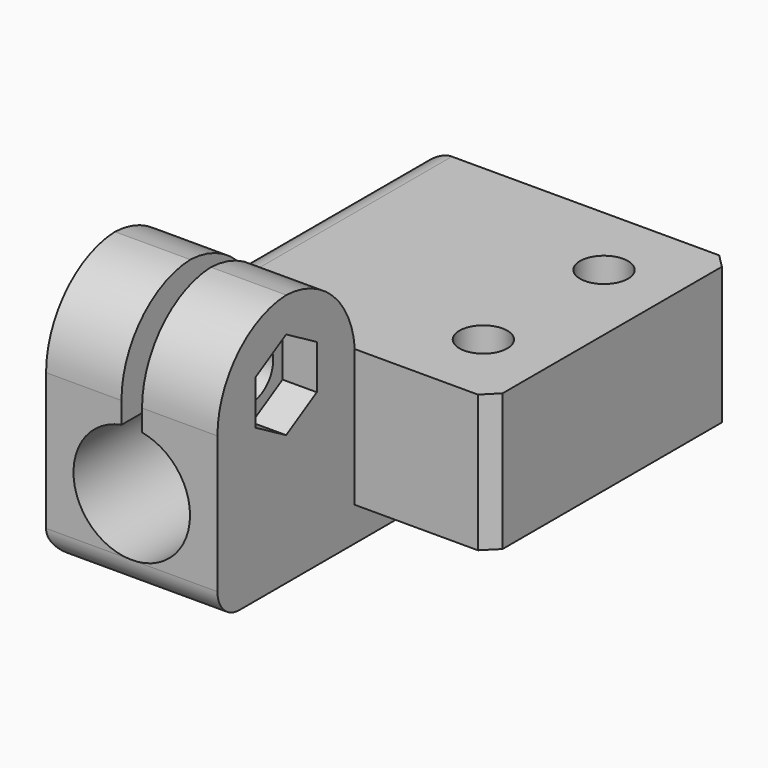
from build123d import *

# Parameters (mm, degrees)
F0_W         = 25
F0_H         = 44
F0_H_2       = 25
F1_DEPTH     = 25
F0_W_2       = 20
F0_R         = 3.5
F2_DEPTH     = 25
F3_R         = 8.5
F4_DEPTH     = 69.001
F5_W         = 11
F5_H         = 25.0466239899
F6_DEPTH     = 12
F5_W_2       = 3
F5_H_2       = 6.9533760101
F7_DEPTH     = 4.1343997347
F9_T1_DEPTH  = 76
F9_T3_DEPTH  = 76
F9_T5_DEPTH  = 75.8074069841
F9_T7_DEPTH  = 75.8074069841
F10_DEPTH    = 5
F8_R         = 3.9
F11_DEPTH    = 25.001
F12_DEPTH    = 25.001
F13_DEPTH    = 5
F14_R        = 3.99999
F15_T1_DEPTH = 30.2867319519


# Not quite as in the source:
# - a fillet or chamfer that OpenCascade refuses, or shapes differently, is made with other operations: its cross-section is extruded or revolved along the edge and cut away or added
# - a fillet or chamfer is up to 0.001 mm smaller than in the source, because OpenCascade refuses the exact size
# - a feature names something its author has since deleted; it is built from what else it names


with BuildPart() as f1:
    # F0 (on Top) → F1 (new body)
    with BuildSketch(Plane.XY):
        Rectangle(F0_W, F0_H)
        with Locations((0, -34.5)):
            Rectangle(F0_W, F0_H_2)
    extrude(amount=F1_DEPTH)

    # F0 (on Top) → F2 (join)
    with BuildSketch(Plane.XY):
        with Locations((22.5, 0)):
            Rectangle(F0_W_2, F0_H)
        with Locations((22.5, -11)):
            Circle(F0_R, mode=Mode.SUBTRACT)
        with Locations((22.5, 11)):
            Circle(F0_R, mode=Mode.SUBTRACT)
    extrude(amount=F2_DEPTH)

    # F3 (on face) → F4 (cut, through all)
    with BuildSketch(Plane.XZ.offset(47)):
        with Locations((0, 12.5)):
            Circle(F3_R)
    extrude(amount=-F4_DEPTH, mode=Mode.SUBTRACT)

    # F5 (on face) → F6 (join)
    with BuildSketch(Plane.XY.offset(25)):
        with Locations((-7, -34.476688005)):
            Rectangle(F5_W, F5_H)
        Polygon((12.5, -22), (12.5, -21.9533760101), (1.5, -21.9533760101), (1.5, -47), (12.5, -47), align=None)
    extrude(amount=F6_DEPTH)

    # F5 (on face) → F7 (cut, through all)
    with BuildSketch(Plane.XY.offset(25)):
        with Locations((0, -34.476688005)):
            Rectangle(F5_W_2, F5_H)
        with Locations((0, -18.476688005)):
            Rectangle(F5_W_2, F5_H_2)
    extrude(amount=-F7_DEPTH, mode=Mode.SUBTRACT)

    # F9: fillet of radius 13 on 4 edges, made by hand

    # F9_s2 → F9_t1 (cut)
    with BuildSketch(Plane.YZ.offset(-45)):
        with BuildLine():
            ThreePointArc((-34, 37), (-43.1923881554, 33.1923881554), (-47, 24))
            Line((-47, 24), (-47, 37))
            Line((-47, 37), (-34, 37))
        make_face()
    extrude(amount=F9_T1_DEPTH, mode=Mode.SUBTRACT)

    # F9_s4 → F9_t3 (cut)
    with BuildSketch(Plane.YZ.offset(-31)):
        with BuildLine():
            ThreePointArc((-34, 37), (-43.1923881554, 33.1923881554), (-47, 24))
            Line((-47, 24), (-47, 37))
            Line((-47, 37), (-34, 37))
        make_face()
    extrude(amount=F9_T3_DEPTH, mode=Mode.SUBTRACT)

    # F9_s6 → F9_t5 (cut)
    with BuildSketch(Plane.YZ.offset(-30.903703492)):
        with BuildLine():
            ThreePointArc((-34.9148574069, 37), (-26.0830965405, 33.5393920142), (-21.9533760101, 25))
            Line((-21.9533760101, 25), (-21.9533760101, 37))
            Line((-21.9533760101, 37), (-34.9148574069, 37))
        make_face()
    extrude(amount=F9_T5_DEPTH, mode=Mode.SUBTRACT)

    # F9_s8 → F9_t7 (cut)
    with BuildSketch(Plane.YZ.offset(-44.903703492)):
        with BuildLine():
            ThreePointArc((-21.9533760101, 25), (-26.0830965405, 33.5393920142), (-34.9148574069, 37))
            Line((-34.9148574069, 37), (-21.9533760101, 37))
            Line((-21.9533760101, 37), (-21.9533760101, 25))
        make_face()
    extrude(amount=F9_T7_DEPTH, mode=Mode.SUBTRACT)

    # F0 (on Top) → F10 (cut)
    with BuildSketch(Plane.XY):
        with Locations((22.5, 0)):
            Rectangle(F0_W_2, F0_H)
        with Locations((22.5, -11)):
            Circle(F0_R, mode=Mode.SUBTRACT)
        with Locations((22.5, 11)):
            Circle(F0_R, mode=Mode.SUBTRACT)
    extrude(amount=F10_DEPTH, mode=Mode.SUBTRACT)

    # F8 (on face) → F11 (cut, through all)
    with BuildSketch(Plane.YZ.offset(12.5)):
        with Locations((-34.476688005, 25.4739885092)):
            Circle(F8_R)
    extrude(amount=-F11_DEPTH, mode=Mode.SUBTRACT)

    # F8 (on face) → F12 (cut, through all)
    with BuildSketch(Plane.YZ.offset(12.5)):
        with Locations((-34.476688005, 25.4739885092)):
            Circle(F8_R)
    extrude(amount=-F12_DEPTH, mode=Mode.SUBTRACT)

    # F8 (on face) → F13 (cut)
    with BuildSketch(Plane.YZ.offset(12.5)):
        Polygon((-40.076688005, 28.7071500166), (-40.076688005, 22.2408270017), (-34.476688005, 19.0076654943), (-28.876688005, 22.2408270017), (-28.876688005, 28.7071500166), (-34.476688005, 31.9403115241), align=None)
        with Locations((-34.476688005, 25.4739885092)):
            Circle(F8_R, mode=Mode.SUBTRACT)
    extrude(amount=-F13_DEPTH, mode=Mode.SUBTRACT)

    # F14 (radius 4 in the source; OpenCascade refuses exactly that, so slightly less here)
    f14_edges = [f1.edges().sort_by_distance(p)[0] for p in [
        (-12.5, -12.5, 0),
        (0, -47, 0),
        (-12.5, 0.023312, 25),
        (0, 22, 0),
        (-12.5, 22, 12.5),
    ]]
    fillet(f14_edges, radius=F14_R)

    # F15: chamfer of 2 on 2 edges, made by hand

    # F15_s2 → F15_t1 (cut)
    with BuildSketch(Plane.XY.offset(-0.1433659759)):
        Polygon((30.5, 22), (32.5, 20), (32.5, 22), align=None)
        Polygon((32.5, -20), (30.5, -22), (32.5, -22), align=None)
    extrude(amount=F15_T1_DEPTH, mode=Mode.SUBTRACT)


solid = f1.part
